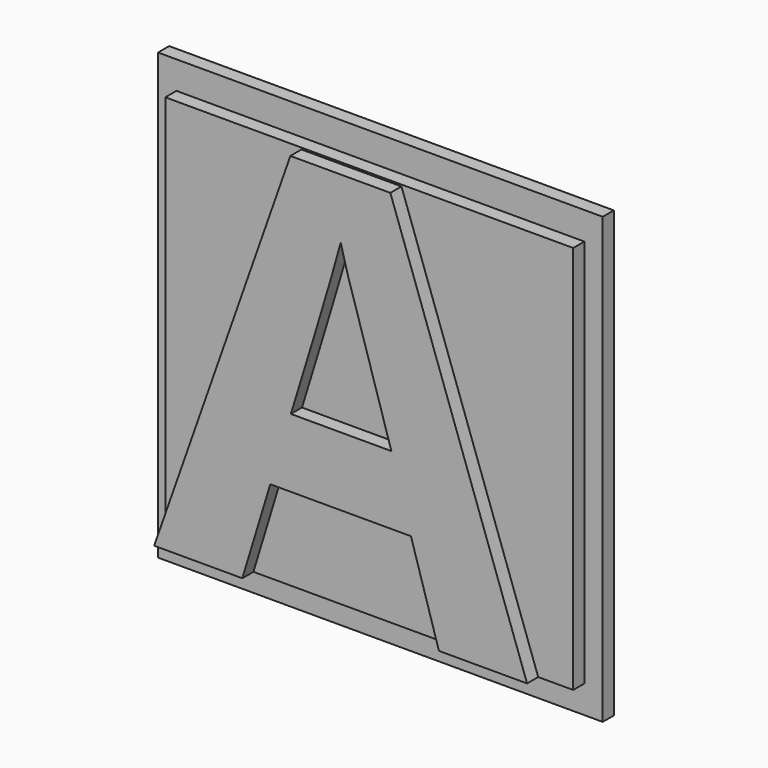
from build123d import *

# Parameters (mm, degrees)
F0_W         = 32
F0_H         = 32
F1_DEPTH     = 1
F2_DEPTH     = 2
F0_TEXT_SIZE = 38.8888888889
F3_DEPTH     = 3


# Not quite as in the source:
# - Text() gives the source's letters only with a copy of the font that has no kerning and outlines rounded to 1/6400 em; it was checked with that copy


with BuildPart() as f1:
    # F0 (on Front) → F1 (new body)
    with BuildSketch(Plane.XZ):
        Rectangle(F0_W, F0_H)
        Polygon((14.6775173611, 14), (14.6775173611, -14), (12.1558159722, -14), (5.8120659722, -14), (-8.3337673611, -14), (-14.6775173611, -14), (-14.6775173611, 14), align=None, mode=Mode.SUBTRACT)
    extrude(amount=F1_DEPTH)

    # F0 (on Front) → F2, piece 2 (join)
    with BuildSketch(Plane.XZ):
        Polygon((12.1558159722, -14), (14.6775173611, -14), (14.6775173611, 14), (-14.6775173611, 14), (-14.6775173611, -14), (-4.8763020833, 13.8784722222), (2.3181423611, 13.8784722222), align=None)
        Polygon((-8.3337673611, -14), (5.8120659722, -14), (3.80078125, -7.3888888889), (-6.3224826389, -7.3888888889), align=None)
    extrude(amount=F2_DEPTH)


with BuildPart() as f2:
    # F0 (on Front) → F2 (new body)
    with BuildSketch(Plane.XZ):
        with BuildLine():
            Line((-4.83984375, -2.4548611111), (2.3910590278, -2.4548611111))
            add(Edge.make_bspline(
                [(2.3910590278, -2.4548611111), (-0.3980034722, 6.5260416667), (-0.7504340278, 7.7048611111)],
                knots=[0, 0, 0, 1, 1, 1], degree=2))
            add(Edge.make_bspline(
                [(-0.7504340278, 7.7048611111), (-1.1028645833, 8.8836805556), (-1.2547743056, 9.5642361111)],
                knots=[0, 0, 0, 1, 1, 1], degree=2))
            add(Edge.make_bspline(
                [(-1.2547743056, 9.5642361111), (-1.8806423611, 7.1336805556), (-4.83984375, -2.4548611111)],
                knots=[0, 0, 0, 1, 1, 1], degree=2))
        make_face()
    extrude(amount=F2_DEPTH)


with BuildPart() as f3:
    # F0 (on Front) → F3 (new body)
    with BuildSketch(Plane.XZ):
        with Locations((-14.6775173611, -14)):
            Text('A', F0_TEXT_SIZE, font='Open Sans', font_style=FontStyle.BOLD, text_align=(TextAlign.LEFT, TextAlign.BOTTOM))
    extrude(amount=F3_DEPTH)


solid = Compound([f1.part, f2.part, f3.part])
